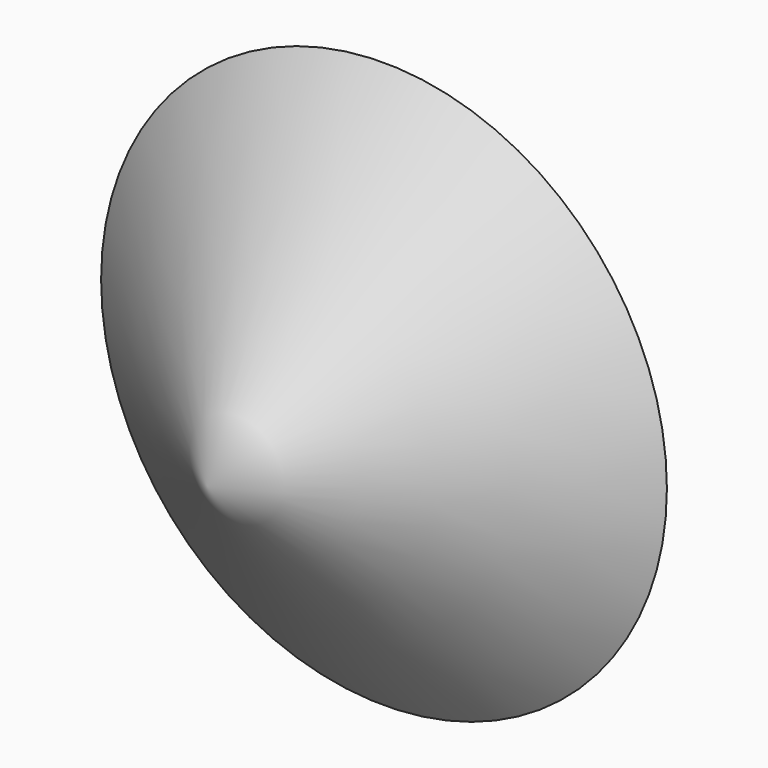
from build123d import *

# Parameters (mm, degrees)
F0_R = 63.5


# Not quite as in the source:
# - an extrude whose draft closes it to a point is written as a loft to that point


with BuildPart() as f1:
    # F0 (on Front) → F1 section 0
    with BuildSketch(Plane.XZ, mode=Mode.PRIVATE) as f1_s0:
        Circle(F0_R)
    loft([f1_s0.sketch, Vertex(0, -49.6116372832, 0)], ruled=True)


solid = f1.part
